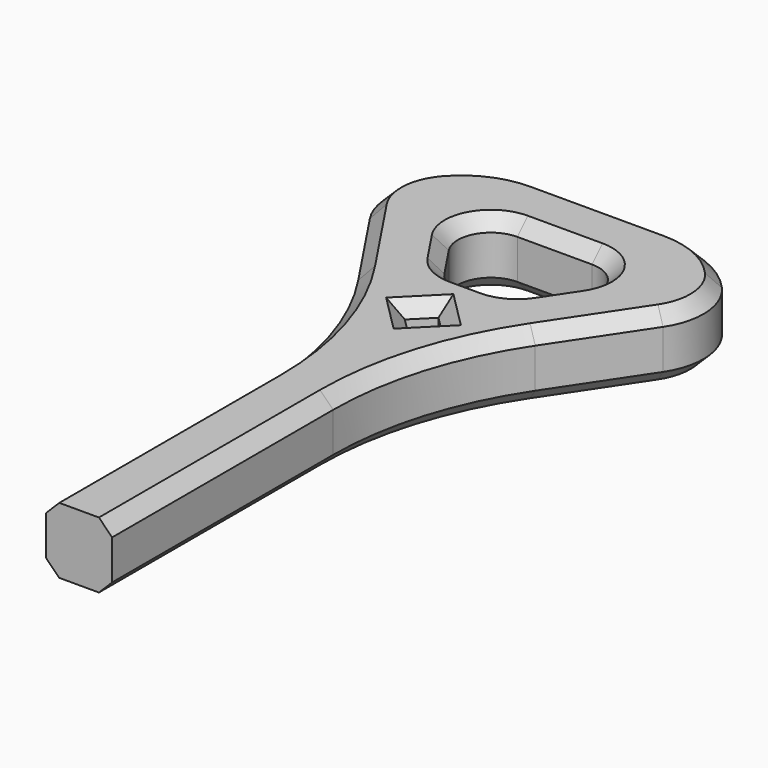
from build123d import *

# Parameters (mm, degrees)
F0_W        = 30
F0_H        = 10
F1_DEPTH    = 10
F2_R        = 5
F3_T1_DEPTH = 84.348882825
F4_R        = 10
F5_R        = 50
F6_SIZE     = 2
F8_DEPTH    = 10.001
F9_SIZE     = 2
F10_DEPTH   = 16
F11_DEPTH   = 25


# Not quite as in the source:
# - a fillet or chamfer that OpenCascade refuses, or shapes differently, is made with other operations: its cross-section is extruded or revolved along the edge and cut away or added


with BuildPart() as f1:
    # F0 (on Top) → F1 (new body)
    with BuildSketch(Plane.XY):
        Polygon((5, 50), (-5, 50), (-15, 65), (-15, 75), (-25, 75), (-25, 61.9722436227), (-5, 31.9722436227), (-5, -50), (5, -50), (5, 31.9722436227), (25, 61.9722436227), (25, 75), (15, 75), (15, 65), align=None)
        with Locations((0, 70)):
            Rectangle(F0_W, F0_H)
    extrude(amount=F1_DEPTH)

    # F2
    f2_edges = [f1.edges().sort_by_distance(p)[0] for p in [
        (15, 65, 5),
        (-15, 65, 5),
        (-5, 50, 5),
        (5, 50, 5),
    ]]
    fillet(f2_edges, radius=F2_R)

    # F3: fillet of radius 15 on 2 edges, made by hand

    # F3_s2 → F3_t1 (cut)
    with BuildSketch(Plane.XY.offset(-37.1744414125)):
        with BuildLine():
            ThreePointArc((-25, 61.9722436227), (-20.0149678844, 71.2823679771), (-10.130223435, 75))
            Line((-10.130223435, 75), (-25, 75))
            Line((-25, 75), (-25, 61.9722436227))
        make_face()
        with BuildLine():
            ThreePointArc((25, 61.9722436227), (20.0149678844, 71.2823679771), (10.130223435, 75))
            Line((10.130223435, 75), (25, 75))
            Line((25, 75), (25, 61.9722436227))
        make_face()
    extrude(amount=F3_T1_DEPTH, mode=Mode.SUBTRACT)

    # F4
    f4_edges = [f1.edges().sort_by_distance(p)[0] for p in [
        (-25, 61.972244, 5),
        (25, 61.972244, 5),
    ]]
    fillet(f4_edges, radius=F4_R)

    # F5
    f5_edges = [f1.edges().sort_by_distance(p)[0] for p in [
        (5, 31.972244, 5),
        (-5, 31.972244, 5),
    ]]
    fillet(f5_edges, radius=F5_R)

    # F6
    f6_edges = [f1.edges().sort_by_distance(p)[0] for p in [
        (0, 65, 10),
        (0, 75, 10),
        (0, 50, 0),
        (0, 75, 0),
    ]]
    chamfer(f6_edges, length=F6_SIZE)

    # F7 (on face) → F8 (cut, through all)
    with BuildSketch(Plane.XY.offset(10)):
        Polygon((0, 37.3431457505), (2.8284271247, 40.1715728753), (0, 43), (-2.8284271247, 40.1715728753), align=None)
    extrude(amount=-F8_DEPTH, mode=Mode.SUBTRACT)

    # F9
    f9_edges = [f1.edges().sort_by_distance(p)[0] for p in [
        (1.414214, 41.585786, 10),
        (-1.414214, 41.585786, 10),
        (1.414214, 38.757359, 10),
        (-1.414214, 38.757359, 10),
        (1.414214, 38.757359, 0),
        (1.414214, 41.585786, 0),
        (-1.414214, 41.585786, 0),
        (-1.414214, 38.757359, 0),
    ]]
    chamfer(f9_edges, length=F9_SIZE)

    # F10 (add): a face of the model
    f10_faces = [f1.faces().sort_by_distance(p)[0] for p in [
        (0, -50, 5),
    ]]
    extrude(f10_faces, amount=-F10_DEPTH)

    # F11 (cut): a face of the model
    f11_faces = [f1.faces().sort_by_distance(p)[0] for p in [
        (0, -50, 5),
    ]]
    extrude(f11_faces, amount=-F11_DEPTH, mode=Mode.SUBTRACT)


solid = f1.part
